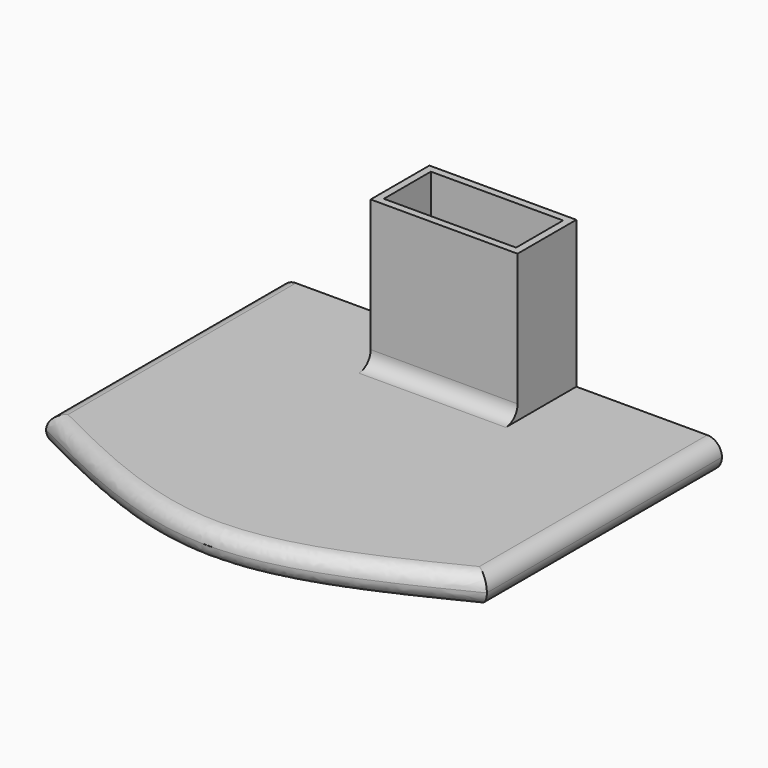
from build123d import *

# Parameters (mm, degrees)
F1_DEPTH = 10
F2_W     = 50
F2_H     = 25
F3_DEPTH = 50
F4_T     = -2.5
F5_R     = 4.999


# Not quite as in the source:
# - a fillet or chamfer is up to 0.001 mm smaller than in the source, because OpenCascade refuses the exact size


with BuildPart() as f1:
    # F0 (on Top) → F1 (new body)
    with BuildSketch(Plane.XY):
        with BuildLine():
            Line((75, 50), (-75, 50))
            Line((-75, 50), (-75, -50))
            add(Edge.make_bspline(
                [(-75, -50), (-50, -62.5487543643), (0, -87.6462630928), (50, -62.5487543643), (75, -50)],
                knots=[0, 0, 0, 0, 0.5, 1, 1, 1, 1], degree=3))
            Line((75, -50), (75, 50))
        make_face()
    extrude(amount=F1_DEPTH)

    # F2 (on face) → F3 (join)
    with BuildSketch(Plane.XY.offset(10)):
        with Locations((0.4496160895, 37.5)):
            Rectangle(F2_W, F2_H)
    extrude(amount=F3_DEPTH)

    # F4
    f4_openings = [f1.faces().sort_by_distance(p)[0] for p in [
        (0.449616, 37.5, 60),
    ]]
    offset(amount=F4_T, openings=f4_openings, kind=Kind.INTERSECTION)

    # F5 (radius 5 in the source; OpenCascade refuses exactly that, so slightly less here)
    f5_edges = [f1.edges().sort_by_distance(p)[0] for p in [
        (0, -75.097509, 10),
        (0, -75.097509, 0),
        (-75, 0, 10),
        (-75, 0, 0),
        (75, 0, 0),
        (75, 0, 10),
        (0.449616, 25, 10),
    ]]
    fillet(f5_edges, radius=F5_R)


solid = f1.part
